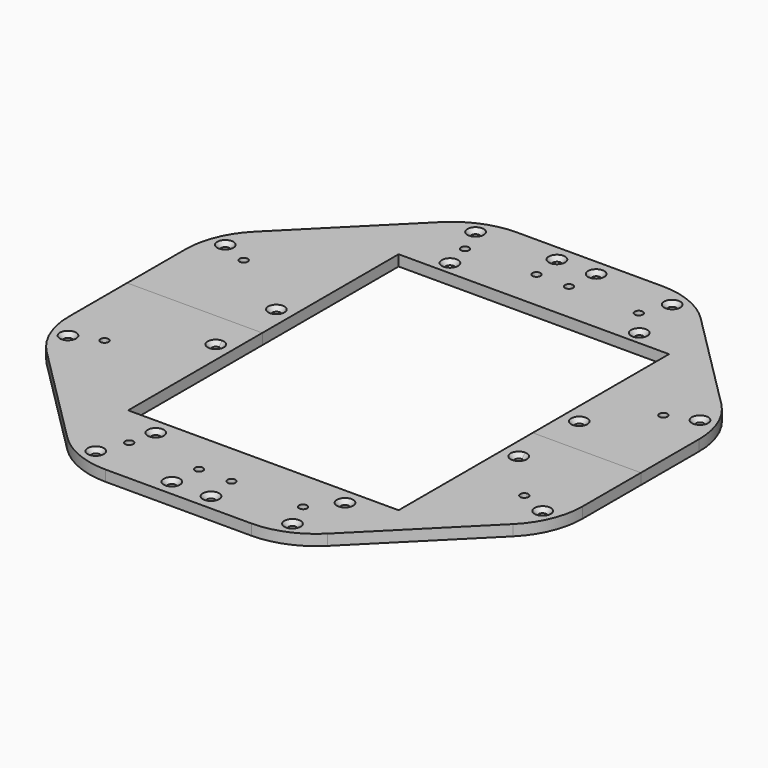
from build123d import *

# Parameters (mm, degrees)
F0_R      = 1.5
F1_DEPTH  = 4
F2_DEPTH  = 4
F3_R      = 30
F3_2_R    = 30
F4_R      = 1.5
F5_DEPTH  = 25
F7_DEPTH  = 25
F8_SIZE   = 1.5
F8_2_SIZE = 1.5


# Not quite as in the source:
# - a feature names something its author has since deleted; it is built from what else it names


with BuildPart() as f1:
    # F0 (on Top) → F1 (new body)
    with BuildSketch(Plane.XY):
        Polygon((0, 0), (95, 0), (95, 39.3502884254), (39.3502884254, 95), (-39.3502884254, 95), (-95, 39.3502884254), (-95, 0), align=None)
        with Locations((-77.6058807309, 32.1454083187)):
            Circle(F0_R, mode=Mode.SUBTRACT)
        with Locations((-87.7685555886, 36.3549260747)):
            Circle(F0_R, mode=Mode.SUBTRACT)
        with Locations((-32.1454083187, 77.6058807309)):
            Circle(F0_R, mode=Mode.SUBTRACT)
        with Locations((-36.3549260747, 87.7685555886)):
            Circle(F0_R, mode=Mode.SUBTRACT)
        with Locations((-6, 78)):
            Circle(F0_R, mode=Mode.SUBTRACT)
        with Locations((-7.25, 89)):
            Circle(F0_R, mode=Mode.SUBTRACT)
        with Locations((77.6058807309, 32.1454083187)):
            Circle(F0_R, mode=Mode.SUBTRACT)
        with Locations((87.7685555886, 36.3549260747)):
            Circle(F0_R, mode=Mode.SUBTRACT)
        with Locations((6, 78)):
            Circle(F0_R, mode=Mode.SUBTRACT)
        with Locations((7.25, 89)):
            Circle(F0_R, mode=Mode.SUBTRACT)
        with Locations((32.1454083187, 77.6058807309)):
            Circle(F0_R, mode=Mode.SUBTRACT)
        with Locations((36.3549260747, 87.7685555886)):
            Circle(F0_R, mode=Mode.SUBTRACT)
    extrude(amount=F1_DEPTH)

    # F3
    f3_edges = [f1.edges().sort_by_distance(p)[0] for p in [
        (95, 39.350288, 2),
        (39.350288, 95, 2),
        (-39.350288, 95, 2),
        (-95, 39.350288, 2),
    ]]
    fillet(f3_edges, radius=F3_R)


with BuildPart() as f2:
    # F0 (on Top) → F2 (new body)
    with BuildSketch(Plane.XY):
        Polygon((-39.3502884254, -95), (39.3502884254, -95), (95, -39.3502884254), (95, 0), (0, 0), (-95, 0), (-95, -39.3502884254), align=None)
        with Locations((-36.3549260747, -87.7685555886)):
            Circle(F0_R, mode=Mode.SUBTRACT)
        with Locations((-32.1454083187, -77.6058807309)):
            Circle(F0_R, mode=Mode.SUBTRACT)
        with Locations((-7.25, -89)):
            Circle(F0_R, mode=Mode.SUBTRACT)
        with Locations((-6, -78)):
            Circle(F0_R, mode=Mode.SUBTRACT)
        with Locations((-87.7685555886, -36.3549260747)):
            Circle(F0_R, mode=Mode.SUBTRACT)
        with Locations((-77.6058807309, -32.1454083187)):
            Circle(F0_R, mode=Mode.SUBTRACT)
        with Locations((7.25, -89)):
            Circle(F0_R, mode=Mode.SUBTRACT)
        with Locations((6, -78)):
            Circle(F0_R, mode=Mode.SUBTRACT)
        with Locations((36.3549260747, -87.7685555886)):
            Circle(F0_R, mode=Mode.SUBTRACT)
        with Locations((32.1454083187, -77.6058807309)):
            Circle(F0_R, mode=Mode.SUBTRACT)
        with Locations((87.7685555886, -36.3549260747)):
            Circle(F0_R, mode=Mode.SUBTRACT)
        with Locations((77.6058807309, -32.1454083187)):
            Circle(F0_R, mode=Mode.SUBTRACT)
    extrude(amount=F2_DEPTH)

    # F3#2
    f3_2_edges = [f2.edges().sort_by_distance(p)[0] for p in [
        (-95, -39.350288, 2),
        (95, -39.350288, 2),
        (-39.350288, -95, 2),
        (39.350288, -95, 2),
    ]]
    fillet(f3_2_edges, radius=F3_2_R)


with BuildPart() as f5_tool:
    # F4 (on face) → F5 (new body)
    with BuildSketch(Plane.XY.offset(4)):
        with Locations((-30, 68)):
            Circle(F4_R)
        with Locations((40, 68)):
            Circle(F4_R)
        with Locations((40, -68)):
            Circle(F4_R)
        with Locations((-30, -68)):
            Circle(F4_R)
    extrude(amount=-F5_DEPTH)


with BuildPart() as f1_1:
    add(f1.part)

    # F5: cut by f5_tool
    add(f5_tool.part, mode=Mode.SUBTRACT)


with BuildPart() as f2_1:
    add(f2.part)

    # F5: cut by f5_tool
    add(f5_tool.part, mode=Mode.SUBTRACT)


with BuildPart() as f7_tool:
    # F6 (on face) → F7 (new body)
    with BuildSketch(Plane.XY.offset(4)):
        with BuildLine():
            ThreePointArc((62.5, 14), (59.9393398282, 15.0606601718), (61, 12.5))
            ThreePointArc((61, 12.5), (62.0606601718, 12.9393398282), (62.5, 14))
        make_face()
        with BuildLine():
            ThreePointArc((-49.5, 14), (-52.0606601718, 15.0606601718), (-51, 12.5))
            ThreePointArc((-51, 12.5), (-49.9393398282, 12.9393398282), (-49.5, 14))
        make_face()
        Polygon((5, 63), (-45, 63), (-45, 0), (0, 0), (55, 0), (55, 63), align=None)
        Polygon((0, 0), (-45, 0), (-45, -62), (55, -62), (55, 0), align=None)
        with BuildLine():
            ThreePointArc((-49.5, -14), (-49.9393398282, -12.9393398282), (-51, -12.5))
            ThreePointArc((-51, -12.5), (-52.0606601718, -15.0606601718), (-49.5, -14))
        make_face()
        with BuildLine():
            ThreePointArc((62.5, -14), (62.0606601718, -12.9393398282), (61, -12.5))
            ThreePointArc((61, -12.5), (59.9393398282, -15.0606601718), (62.5, -14))
        make_face()
    extrude(amount=-F7_DEPTH)


with BuildPart() as f1_2:
    add(f1_1.part)

    # F7: cut by f7_tool
    add(f7_tool.part, mode=Mode.SUBTRACT)

    # F8
    f8_edges = [f1_2.edges().sort_by_distance(p)[0] for p in [
        (-31.5, 68, 4),
        (38.5, 68, 4),
        (-89.268556, 36.354926, 4),
        (-37.854926, 87.768556, 4),
        (-8.75, 89, 4),
        (5.75, 89, 4),
        (34.854926, 87.768556, 4),
        (86.268556, 36.354926, 4),
        (-79.105881, 32.145408, 0),
        (76.105881, 32.145408, 0),
        (30.645408, 77.605881, 0),
        (4.5, 78, 0),
        (-7.5, 78, 0),
        (-33.645408, 77.605881, 0),
        (-52.5, 14, 4),
        (59.5, 14, 4),
    ]]
    chamfer(f8_edges, length=F8_SIZE)


with BuildPart() as f2_2:
    add(f2_1.part)

    # F7: cut by f7_tool
    add(f7_tool.part, mode=Mode.SUBTRACT)

    # F8#2
    f8_2_edges = [f2_2.edges().sort_by_distance(p)[0] for p in [
        (-31.5, -68, 4),
        (38.5, -68, 4),
        (34.854926, -87.768556, 4),
        (5.75, -89, 4),
        (-8.75, -89, 4),
        (-37.854926, -87.768556, 4),
        (-89.268556, -36.354926, 4),
        (86.268556, -36.354926, 4),
        (-79.105881, -32.145408, 0),
        (-33.645408, -77.605881, 0),
        (-7.5, -78, 0),
        (4.5, -78, 0),
        (30.645408, -77.605881, 0),
        (76.105881, -32.145408, 0),
        (-52.5, -14, 4),
        (59.5, -14, 4),
    ]]
    chamfer(f8_2_edges, length=F8_2_SIZE)


solid = Compound([f1_2.part, f2_2.part])
